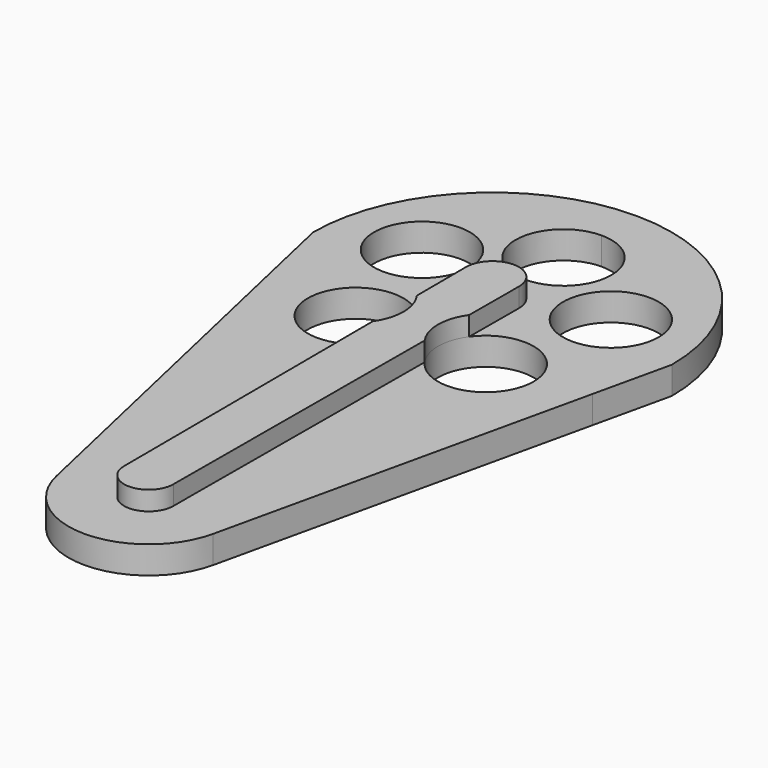
from build123d import *

# Parameters (mm, degrees)
F0_R     = 10.16
F1_DEPTH = 5.842
F2_DEPTH = 5.842
F4_DEPTH = 4.064


# Not quite as in the source:
# - after a boolean that leaves OpenCascade's solid faulty, fix() repairs it
# - ends of sketch curves that miss each other by under 0.0002 mm in the source are joined


with BuildPart() as f1:
    # F0 (on Top) → F1 (new body)
    with BuildSketch(Plane.XY):
        with BuildLine():
            Line((0, 28.9974835998), (0, 38.1))
            ThreePointArc((0, 38.1), (-26.9407683632, 26.9407683632), (-38.1, 0))
            Line((-38.1, 0), (-34.39917941, -16.3800627568))
            ThreePointArc((-34.39917941, -16.3800627568), (-20.3412095138, -32.2156048448), (0, -38.1))
            Line((0, -38.1), (0, 8.6774835998))
            ThreePointArc((0, 8.6774835998), (-10.16, 18.8374835998), (0, 28.9974835998))
        make_face()
        with Locations((-13.8204852119, -19.0573949367)):
            Circle(F0_R, mode=Mode.SUBTRACT)
        with Locations((-20.0619921088, 6.3544651493)):
            Circle(F0_R, mode=Mode.SUBTRACT)
        with BuildLine():
            Line((34.39917941, -16.3800627568), (38.1, 0))
            ThreePointArc((38.1, 0), (26.9407683632, 26.9407683632), (0, 38.1))
            Line((0, 38.1), (0, 28.9974835998))
            ThreePointArc((0, 28.9974835998), (7.1842048969, 26.0216884966), (10.16, 18.8374835998))
            ThreePointArc((10.16, 18.8374835998), (7.1842048969, 11.6532787029), (0, 8.6774835998))
            Line((0, 8.6774835998), (0, -38.1))
            ThreePointArc((0, -38.1), (20.3412095138, -32.2156048448), (34.39917941, -16.3800627568))
        make_face()
        with Locations((13.8204852119, -19.0573949367)):
            Circle(F0_R, mode=Mode.SUBTRACT)
        with Locations((20.0619921088, 6.3544651493)):
            Circle(F0_R, mode=Mode.SUBTRACT)
    extrude(amount=F1_DEPTH)

    # F0 (on Top) → F2 (join)
    with BuildSketch(Plane.XY):
        with BuildLine():
            Line((16.6278202087, -95.0372070074), (34.39917941, -16.3800627568))
            ThreePointArc((34.39917941, -16.3800627568), (20.3412095138, -32.2156048448), (0, -38.1))
            ThreePointArc((0, -38.1), (-20.3412095138, -32.2156048448), (-34.39917941, -16.3800627568))
            Line((-34.39917941, -16.3800627568), (-16.6278202087, -95.0372070074))
            ThreePointArc((-16.6278202087, -95.0372070074), (0, -108.3273427039), (16.6278202087, -95.0372070074))
        make_face()
    extrude(amount=F2_DEPTH)

    # F3 (on face) → F4 (join)
    with BuildSketch(Plane.XY.offset(5.842)):
        with BuildLine():
            Line((5.5590673185, -13.1434644002), (5.6142329033, 0))
            ThreePointArc((5.6142329033, 0), (0, 5.6142329033), (-5.6142329033, 0))
            Line((-5.6142329033, 0), (-5.5590673185, -13.1434644002))
            ThreePointArc((-5.5590673185, -13.1434644002), (-4.1467680929, -15.9517875723), (-3.6604852119, -19.0573949367))
            ThreePointArc((-3.6604852119, -19.0573949367), (-4.1338185981, -22.1223728994), (-5.5097155096, -24.9017688941))
            Line((-5.5097155096, -24.9017688941), (-5.2310197557, -91.3023650429))
            ThreePointArc((-5.2310197557, -91.3023650429), (-0.0109778096, -86.0493551595), (5.2310658314, -91.280409472))
            Line((5.2310658314, -91.280409472), (5.5097155096, -24.9017688941))
            ThreePointArc((5.5097155096, -24.9017688941), (3.660574702, -19.014751887), (5.5590673185, -13.1434644002))
        make_face()
        with BuildLine():
            ThreePointArc((5.2310197557, -91.3023650429), (5.2310543125, -91.2913872816), (5.2310658314, -91.280409472))
            ThreePointArc((5.2310658314, -91.280409472), (-0.0109778096, -86.0493551595), (-5.2310197557, -91.3023650429))
            ThreePointArc((-5.2310197557, -91.3023650429), (0, -96.5114753034), (5.2310197557, -91.3023650429))
        make_face()
    extrude(amount=F4_DEPTH)

    add(f1.part.fix(), mode=Mode.REPLACE)


solid = f1.part
